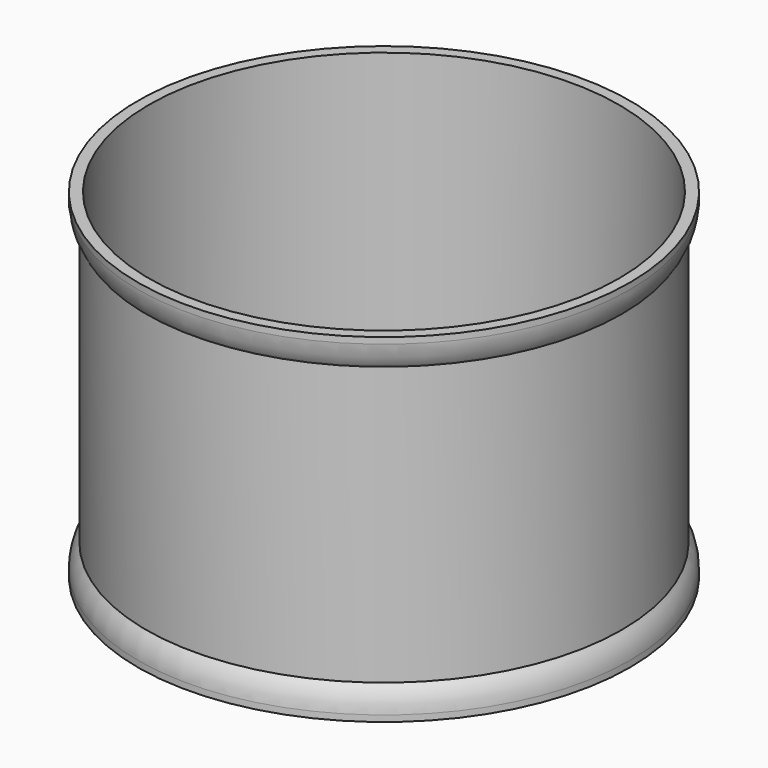
from build123d import *

# Parameters (mm, degrees)
F0_R     = 37.235
F0_R_2   = 35.57
F1_DEPTH = 4.6
F2_R     = 36
F2_R_2   = 35.57
F3_DEPTH = 42.07
F4_R     = 37.235
F4_R_2   = 35.57
F5_DEPTH = 4.6


# Not quite as in the source:
# - a fillet or chamfer that OpenCascade refuses, or shapes differently, is made with other operations: its cross-section is extruded or revolved along the edge and cut away or added


with BuildPart() as f1:
    # F0 (on Top) → F1 (new body)
    with BuildSketch(Plane.XY):
        Circle(F0_R)
        Circle(F0_R_2, mode=Mode.SUBTRACT)
    extrude(amount=F1_DEPTH)

    # F2 (on face) → F3 (join)
    with BuildSketch(Plane.XY.offset(4.6)):
        Circle(F2_R)
        Circle(F2_R_2, mode=Mode.SUBTRACT)
    extrude(amount=F3_DEPTH)

    # F4 (on face) → F5 (join)
    with BuildSketch(Plane.XY.offset(46.67)):
        Circle(F4_R)
        Circle(F4_R_2, mode=Mode.SUBTRACT)
    extrude(amount=F5_DEPTH)

    # F6: fillet of radius 6.0355339059 on 2 edges, made by hand

    # F6_s1 → F6_t2 (revolve, cut)
    with BuildSketch(Plane.XZ):
        with BuildLine():
            ThreePointArc((37.235, 0.9417840759), (36.9179210727, 2.8723130673), (36, 4.6))
            Line((36, 4.6), (37.235, 4.6))
            Line((37.235, 4.6), (37.235, 0.9417840759))
        make_face()
    revolve(axis=Axis((0, 0, 4.6), (0, 0, 1)), mode=Mode.SUBTRACT)

    # F6_s3 → F6_t4 (revolve, cut)
    with BuildSketch(Plane.XZ):
        with BuildLine():
            ThreePointArc((36, 46.67), (36.9179210727, 48.3976869327), (37.235, 50.3282159241))
            Line((37.235, 50.3282159241), (37.235, 46.67))
            Line((37.235, 46.67), (36, 46.67))
        make_face()
    revolve(axis=Axis((0, 0, 46.67), (0, 0, 1)), mode=Mode.SUBTRACT)


solid = f1.part
